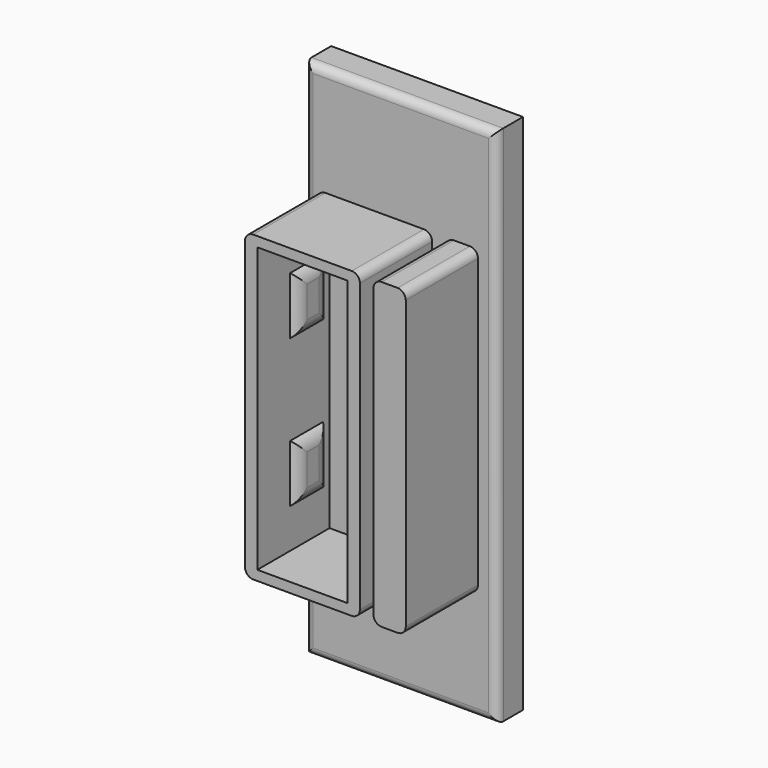
from build123d import *

# Parameters (mm, degrees)
F0_W        = 10.795
F0_H        = 25.4
F1_DEPTH    = 2.54
F2_W        = 8.89
F2_H        = 23.495
F2_W_2      = 6.985
F2_H_2      = 21.971
F3_DEPTH    = 6.985
F4_W        = 3.175
F4_H        = 4.445
F5_DEPTH    = 0.5
F6_W        = 3.175
F6_H        = 4.445
F7_DEPTH    = 0.5
F8_T1_DEPTH = 5.6998762346
F8_T3_DEPTH = 9.4947524692
F8_T5_DEPTH = 9.4947524692
F9_W        = 10.795
F9_H        = 7.5
F10_DEPTH   = 2.54
F11_W       = 2.5
F11_H       = 23.495
F12_DEPTH   = 6.985
F13_R       = 0.635


# Not quite as in the source:
# - a fillet or chamfer that OpenCascade refuses, or shapes differently, is made with other operations: its cross-section is extruded or revolved along the edge and cut away or added


with BuildPart() as f1:
    # F0 (on Front) → F1 (new body)
    with BuildSketch(Plane.XZ):
        with Locations((5.3975, -12.7)):
            Rectangle(F0_W, F0_H)
    extrude(amount=F1_DEPTH)

    # F2 (on face) → F3 (join)
    with BuildSketch(Plane.XZ.offset(2.54)):
        with Locations((5.3975, -12.7)):
            Rectangle(F2_W, F2_H)
        with Locations((5.3975, -12.7)):
            Rectangle(F2_W_2, F2_H_2, mode=Mode.SUBTRACT)
    extrude(amount=F3_DEPTH)

    # F4 (on face) → F5 (join)
    with BuildSketch(Plane.YZ.offset(1.905)):
        with Locations((-4.7625, -6.985)):
            Rectangle(F4_W, F4_H)
        with Locations((-4.7625, -18.415)):
            Rectangle(F4_W, F4_H)
    extrude(amount=F5_DEPTH)

    # F6 (on face) → F7 (join)
    with BuildSketch(Plane(origin=(8.89, 0, 0), x_dir=(0, -1, 0), z_dir=(-1, 0, 0))):
        with Locations((4.7625, -6.985)):
            Rectangle(F6_W, F6_H)
        with Locations((4.7625, -18.415)):
            Rectangle(F6_W, F6_H)
    extrude(amount=F7_DEPTH)

    # F8: fillet of radius 1.27 on 16 edges, made by hand

    # F8_s2 → F8_t1 (cut)
    with BuildSketch(Plane.XZ.offset(3.175)):
        with BuildLine():
            ThreePointArc((1.905, -16.1925), (2.273156404, -16.6389791104), (2.405, -17.2024504938))
            Line((2.405, -17.2024504938), (2.405, -16.1925))
            Line((2.405, -16.1925), (1.905, -16.1925))
        make_face()
        with BuildLine():
            ThreePointArc((1.905, -20.6375), (2.273156404, -20.1910208896), (2.405, -19.6275495062))
            Line((2.405, -19.6275495062), (2.405, -20.6375))
            Line((2.405, -20.6375), (1.905, -20.6375))
        make_face()
        with BuildLine():
            ThreePointArc((1.905, -4.7625), (2.273156404, -5.2089791104), (2.405, -5.7724504938))
            Line((2.405, -5.7724504938), (2.405, -4.7625))
            Line((2.405, -4.7625), (1.905, -4.7625))
        make_face()
        with BuildLine():
            ThreePointArc((1.905, -9.2075), (2.273156404, -8.7610208896), (2.405, -8.1975495062))
            Line((2.405, -8.1975495062), (2.405, -9.2075))
            Line((2.405, -9.2075), (1.905, -9.2075))
        make_face()
        with BuildLine():
            ThreePointArc((8.89, -4.7625), (8.521843596, -5.2089791104), (8.39, -5.7724504938))
            Line((8.39, -5.7724504938), (8.39, -4.7625))
            Line((8.39, -4.7625), (8.89, -4.7625))
        make_face()
        with BuildLine():
            ThreePointArc((8.89, -9.2075), (8.521843596, -8.7610208896), (8.39, -8.1975495062))
            Line((8.39, -8.1975495062), (8.39, -9.2075))
            Line((8.39, -9.2075), (8.89, -9.2075))
        make_face()
        with BuildLine():
            ThreePointArc((8.89, -16.1925), (8.521843596, -16.6389791104), (8.39, -17.2024504938))
            Line((8.39, -17.2024504938), (8.39, -16.1925))
            Line((8.39, -16.1925), (8.89, -16.1925))
        make_face()
        with BuildLine():
            ThreePointArc((8.89, -20.6375), (8.521843596, -20.1910208896), (8.39, -19.6275495062))
            Line((8.39, -19.6275495062), (8.39, -20.6375))
            Line((8.39, -20.6375), (8.89, -20.6375))
        make_face()
    extrude(amount=F8_T1_DEPTH, mode=Mode.SUBTRACT)

    # F8_s4 → F8_t3 (cut)
    with BuildSketch(Plane.XY.offset(-23.1623762346)):
        with BuildLine():
            ThreePointArc((1.905, -6.35), (2.273156404, -5.9035208896), (2.405, -5.3400495062))
            Line((2.405, -5.3400495062), (2.405, -6.35))
            Line((2.405, -6.35), (1.905, -6.35))
        make_face()
        with BuildLine():
            ThreePointArc((1.905, -3.175), (2.273156404, -3.6214791104), (2.405, -4.1849504938))
            Line((2.405, -4.1849504938), (2.405, -3.175))
            Line((2.405, -3.175), (1.905, -3.175))
        make_face()
        with BuildLine():
            ThreePointArc((8.89, -3.175), (8.521843596, -3.6214791104), (8.39, -4.1849504938))
            Line((8.39, -4.1849504938), (8.39, -3.175))
            Line((8.39, -3.175), (8.89, -3.175))
        make_face()
        with BuildLine():
            ThreePointArc((8.89, -6.35), (8.521843596, -5.9035208896), (8.39, -5.3400495062))
            Line((8.39, -5.3400495062), (8.39, -6.35))
            Line((8.39, -6.35), (8.89, -6.35))
        make_face()
    extrude(amount=F8_T3_DEPTH, mode=Mode.SUBTRACT)

    # F8_s6 → F8_t5 (cut)
    with BuildSketch(Plane.XY.offset(-11.7323762346)):
        with BuildLine():
            ThreePointArc((1.905, -6.35), (2.273156404, -5.9035208896), (2.405, -5.3400495062))
            Line((2.405, -5.3400495062), (2.405, -6.35))
            Line((2.405, -6.35), (1.905, -6.35))
        make_face()
        with BuildLine():
            ThreePointArc((1.905, -3.175), (2.273156404, -3.6214791104), (2.405, -4.1849504938))
            Line((2.405, -4.1849504938), (2.405, -3.175))
            Line((2.405, -3.175), (1.905, -3.175))
        make_face()
        with BuildLine():
            ThreePointArc((8.89, -3.175), (8.521843596, -3.6214791104), (8.39, -4.1849504938))
            Line((8.39, -4.1849504938), (8.39, -3.175))
            Line((8.39, -3.175), (8.89, -3.175))
        make_face()
        with BuildLine():
            ThreePointArc((8.89, -6.35), (8.521843596, -5.9035208896), (8.39, -5.3400495062))
            Line((8.39, -5.3400495062), (8.39, -6.35))
            Line((8.39, -6.35), (8.89, -6.35))
        make_face()
    extrude(amount=F8_T5_DEPTH, mode=Mode.SUBTRACT)

    # F9 (on Front) → F10 (join)
    with BuildSketch(Plane.XZ):
        with Locations((5.3975, 3.75)):
            Rectangle(F9_W, F9_H)
        Polygon((10.795, 7.5), (10.795, 0), (10.795, -25.4), (10.795, -32.9), (14.8425, -32.9), (14.8425, 7.5), align=None)
        with Locations((5.3975, -29.15)):
            Rectangle(F9_W, F9_H)
    extrude(amount=F10_DEPTH)

    # F11 (on face) → F12 (join)
    with BuildSketch(Plane.XZ.offset(2.54)):
        with Locations((12.1425, -12.7)):
            Rectangle(F11_W, F11_H)
    extrude(amount=F12_DEPTH)

    # F13
    f13_edges = [f1.edges().sort_by_distance(p)[0] for p in [
        (0.9525, -6.0325, -0.9525),
        (9.8425, -6.0325, -0.9525),
        (9.8425, -6.0325, -24.4475),
        (0.9525, -6.0325, -24.4475),
        (0, -2.54, -12.7),
        (10.8925, -6.0325, -24.4475),
        (13.3925, -6.0325, -24.4475),
        (10.8925, -6.0325, -0.9525),
        (13.3925, -6.0325, -0.9525),
        (14.8425, -2.54, -12.7),
        (7.42125, -2.54, -32.9),
        (7.42125, -2.54, 7.5),
    ]]
    fillet(f13_edges, radius=F13_R)


solid = f1.part
